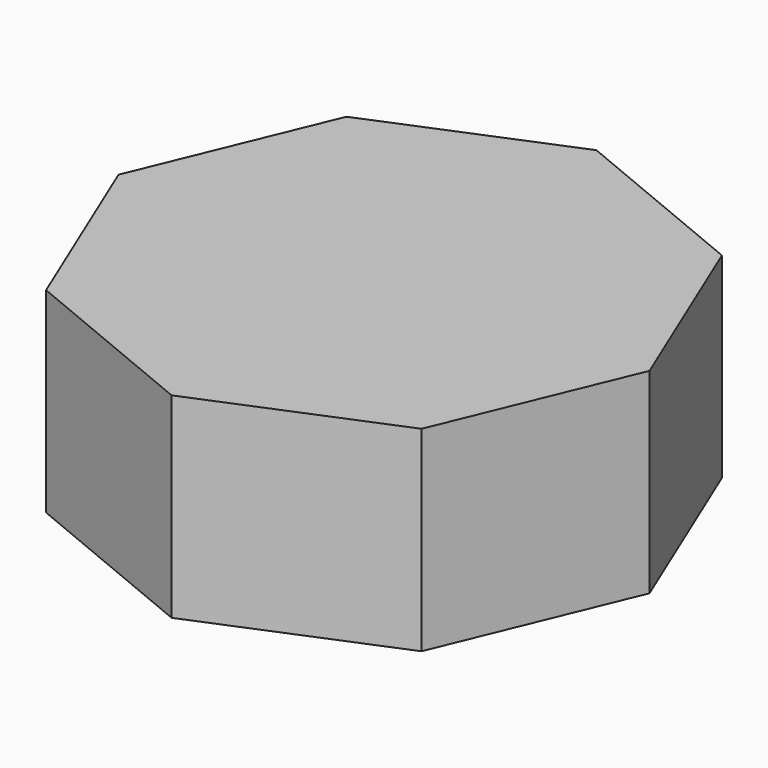
from build123d import *

# Parameters (mm, degrees)
F0_R     = 11.2476084484
F1_DEPTH = 14.478


# Not quite as in the source:
# - a feature of the source that left no trace in its solid (it failed there, or was rolled back) is left out


with BuildPart() as f1:
    # F0 (on Top) → F1 (new body)
    with BuildSketch(Plane.XY):
        Polygon((13.876531439, -13.876531439), (19.6243789597, 0), (13.876531439, 13.876531439), (0, 19.6243789597), (-13.876531439, 13.876531439), (-19.6243789597, 0), (-13.876531439, -13.876531439), (0, -19.6243789597), align=None)
        Circle(F0_R, mode=Mode.SUBTRACT)
        Circle(F0_R)
    extrude(amount=F1_DEPTH)


solid = f1.part
